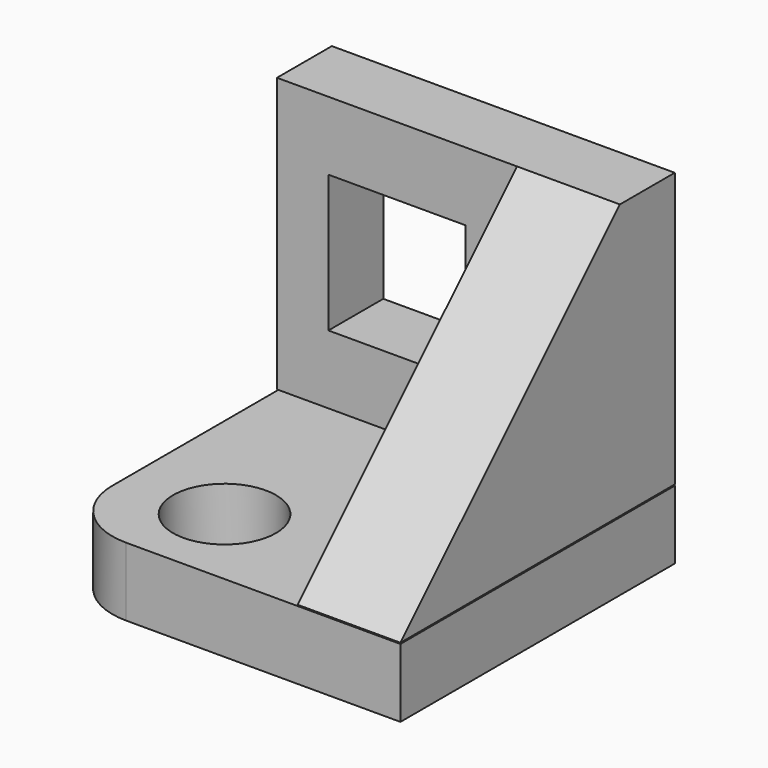
from build123d import *

# Parameters (mm, degrees)
F0_W      = 100
F0_H      = 100
F1_DEPTH  = 20
F2_W      = 100
F2_H      = 80
F3_DEPTH  = 20
F4_R      = 15
F5_DEPTH  = 22
F6_W      = 80
F6_H      = 80
F7_DEPTH  = 30
F8_SIZE   = 79.99999
F9_R      = 20
F10_W     = 40
F10_H     = 40
F11_DEPTH = 25


# Not quite as in the source:
# - a fillet or chamfer is up to 0.001 mm smaller than in the source, because OpenCascade refuses the exact size


with BuildPart() as f1:
    # F0 (on Top) → F1 (new body)
    with BuildSketch(Plane.XY):
        with Locations((-50, -50)):
            Rectangle(F0_W, F0_H)
    extrude(amount=F1_DEPTH)

    # F4 (on face) → F5 (cut)
    with BuildSketch(Plane.XY.offset(20)):
        with Locations((-71.2947770953, -75)):
            Circle(F4_R)
    extrude(amount=-F5_DEPTH, mode=Mode.SUBTRACT)

    # F9
    f9_edges = [f1.edges().sort_by_distance(p)[0] for p in [
        (-100, -100, 10),
    ]]
    fillet(f9_edges, radius=F9_R)


with BuildPart() as f3:
    # F2 (on Front) → F3 (new body)
    with BuildSketch(Plane.XZ):
        with Locations((-50, 60.3316903863)):
            Rectangle(F2_W, F2_H)
    extrude(amount=F3_DEPTH)

    # F6 (on face) → F7 (join)
    with BuildSketch(Plane.YZ):
        with Locations((-60, 60.3316903863)):
            Rectangle(F6_W, F6_H)
    extrude(amount=-F7_DEPTH)

    # F8 (size 80 in the source; OpenCascade refuses exactly that, so slightly less here)
    f8_edges = [f3.edges().sort_by_distance(p)[0] for p in [
        (-15, -100, 100.33169),
    ]]
    chamfer(f8_edges, length=F8_SIZE)

    # F10 (on face) → F11 (cut)
    with BuildSketch(Plane.XZ.offset(20)):
        with Locations((-65, 60.3316903863)):
            Rectangle(F10_W, F10_H)
    extrude(amount=-F11_DEPTH, mode=Mode.SUBTRACT)


solid = Compound([f1.part, f3.part])
